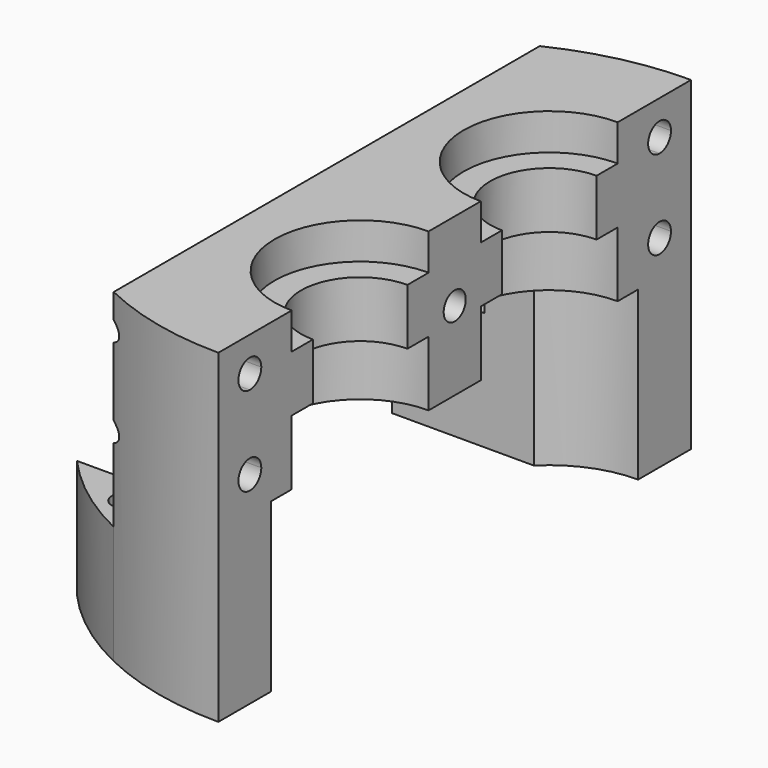
from build123d import *

# Parameters (mm, degrees)
F1_DEPTH      = 33
F3_DEPTH      = 12
F6_DEPTH      = 35.361679775
F7_R          = 6
F8_DEPTH      = 17.001
F9_W          = 4.1692499071
F9_H          = 40.0000885129
F10_DEPTH     = 8
F11_R         = 1.4
F12_DEPTH     = 35.361679775
F10_FACE2_W   = 4.1692499071
F10_FACE2_H   = 40.0000885129
F14_DEPTH     = 33.001
F15_W         = 2.69
F15_H         = 3.69
F15_H_2       = 6.6
F17_W         = 2.69
F17_H         = 6.6
F17_H_2       = 3.69
F20_DEPTH     = 33.001
F21_TEXT_SIZE = 11.6276503023
F22_DEPTH     = 1.69
F24_DEPTH     = 22.361679775


# Not quite as in the source:
# - Text() gives the source's letters only with a copy of the font that has no kerning and outlines rounded to 1/6400 em; it was checked with that copy


with BuildPart() as f1:
    # F0 (on Top) → F1 (new body)
    with BuildSketch(Plane.XY):
        with BuildLine():
            Line((-13, 27.0370116692), (13, 27.0370116692))
            ThreePointArc((13, 27.0370116692), (0, 30), (-13, 27.0370116692))
        make_face()
        with BuildLine():
            ThreePointArc((-13, -27.0370116692), (0, -30), (13, -27.0370116692))
            Line((13, -27.0370116692), (-13, -27.0370116692))
        make_face()
        with BuildLine():
            Line((13, -12), (6, -12))
            ThreePointArc((6, -12), (0, -18), (-6, -12))
            Line((-6, -12), (-13, -12))
            Line((-13, -12), (-13, -27.0370116692))
            Line((-13, -27.0370116692), (13, -27.0370116692))
            Line((13, -27.0370116692), (13, -12))
        make_face()
        with BuildLine():
            ThreePointArc((-6, -12), (0, -6), (6, -12))
            Line((6, -12), (13, -12))
            Line((13, -12), (13, 12))
            Line((13, 12), (6, 12))
            ThreePointArc((6, 12), (0, 6), (-6, 12))
            Line((-6, 12), (-13, 12))
            Line((-13, 12), (-13, -12))
            Line((-13, -12), (-6, -12))
        make_face()
        with BuildLine():
            Line((6, 12), (13, 12))
            Line((13, 12), (13, 27.0370116692))
            Line((13, 27.0370116692), (-13, 27.0370116692))
            Line((-13, 27.0370116692), (-13, 12))
            Line((-13, 12), (-6, 12))
            ThreePointArc((-6, 12), (0, 18), (6, 12))
        make_face()
    extrude(amount=F1_DEPTH)

    # F2 (on Top) → F3 (join)
    with BuildSketch(Plane.XY):
        with BuildLine():
            Line((-12.8831444308, 20), (22.360679775, 20))
            ThreePointArc((22.360679775, 20), (0, 30), (-22.360679775, 20))
            Line((-22.360679775, 20), (-12.8831444308, 20))
        make_face()
        with BuildLine():
            ThreePointArc((-22.360679775, -20), (0, -30), (22.360679775, -20))
            Line((22.360679775, -20), (-12.8831444308, -20))
            Line((-12.8831444308, -20), (-22.360679775, -20))
        make_face()
    extrude(amount=F3_DEPTH)

    # F5 (on face) → F6 (cut, through all)
    with BuildSketch(Plane(origin=(-13, 0, 0), x_dir=(0, -1, 0), z_dir=(-1, 0, 0))):
        Polygon((-20, 12), (-20, 0), (20, 0), (20, 12), (20, 17), (-20, 17), align=None)
    extrude(amount=-F6_DEPTH, mode=Mode.SUBTRACT)

    # F7 (on face) → F8 (cut, through all)
    with BuildSketch(Plane(origin=(0, 0, 17), x_dir=(1, 0, 0), z_dir=(0, 0, -1))):
        with BuildLine():
            ThreePointArc((-7.9664358404, 20), (-4.3314569928, 1.5739470403), (11.29, 12))
            ThreePointArc((11.29, 12), (10.4260529597, 16.3314569928), (7.9664358404, 20))
            Line((7.9664358404, 20), (-7.9664358404, 20))
        make_face()
        with Locations((0, 12)):
            Circle(F7_R, mode=Mode.SUBTRACT)
        with Locations((0, -12)):
            Circle(F7_R)
        with Locations((0, 12)):
            Circle(F7_R)
        with BuildLine():
            Line((-7.9664358404, 20), (7.9664358404, 20))
            ThreePointArc((7.9664358404, 20), (0, 23.29), (-7.9664358404, 20))
        make_face()
        with BuildLine():
            ThreePointArc((-7.9664358404, -20), (0, -23.29), (7.9664358404, -20))
            Line((7.9664358404, -20), (-7.9664358404, -20))
        make_face()
    extrude(amount=F8_DEPTH, mode=Mode.SUBTRACT)

    # F9 (on face) → F10 (join)
    with BuildSketch(Plane.XY.offset(33)):
        with Locations((10.915457271, 0)):
            Rectangle(F9_W, F9_H)
    extrude(amount=F10_DEPTH)

    # F11 (on face) → F12 (cut, through all)
    with BuildSketch(Plane.YZ.offset(13)):
        with Locations((-16.0000442564, 36)):
            Circle(F11_R)
        with Locations((15.9999557436, 36)):
            Circle(F11_R)
    extrude(amount=-F12_DEPTH, mode=Mode.SUBTRACT)

    # F4 (on face) + F10_face2 (on face) → F14 (cut, through all)
    with BuildSketch(Plane.XY.offset(33)):
        with BuildLine():
            Line((0, 36.6020798683), (0, 35.8893685043))
            Line((0, 35.8893685043), (0, 33.0385304987))
            Line((0, 33.0385304987), (0, 30))
            ThreePointArc((0, 30), (6.6666952054, 29.2498747867), (13, 27.0370116692))
            Line((13, 27.0370116692), (13, -27.0370116692))
            ThreePointArc((13, -27.0370116692), (6.6666952054, -29.2498747867), (0, -30))
            Line((0, -30), (0, -37.9473641515))
            Line((0, -37.9473641515), (28.5907108337, -37.9473641515))
            Line((28.5907108337, -37.9473641515), (28.5907108337, 36.6020798683))
            Line((28.5907108337, 36.6020798683), (0, 36.6020798683))
        make_face()
        with BuildLine():
            ThreePointArc((13, 27.0370116692), (6.6666952054, 29.2498747867), (0, 30))
            Line((0, 30), (0, 18))
            ThreePointArc((0, 18), (4.2426406871, 16.2426406871), (6, 12))
            ThreePointArc((6, 12), (4.2426406871, 7.7573593129), (0, 6))
            Line((0, 6), (0, -6))
            ThreePointArc((0, -6), (4.2426406871, -7.7573593129), (6, -12))
            ThreePointArc((6, -12), (4.2426406871, -16.2426406871), (0, -18))
            Line((0, -18), (0, -30))
            ThreePointArc((0, -30), (6.6666952054, -29.2498747867), (13, -27.0370116692))
            Line((13, -27.0370116692), (13, 27.0370116692))
        make_face()
    with BuildSketch(Plane(origin=(10.915457271, 0, 41), x_dir=(1, 0, 0), z_dir=(0, 0, 1))):
        Rectangle(F10_FACE2_W, F10_FACE2_H)
    extrude(amount=-F14_DEPTH, mode=Mode.SUBTRACT)

    # F15 (on face) → F16 (revolve, cut)
    with BuildSketch(Plane.YZ):
        with Locations((19.345, 31.155)):
            Rectangle(F15_W, F15_H)
        with Locations((19.345, 20.3)):
            Rectangle(F15_W, F15_H_2)
    revolve(axis=Axis((0, 12, 24.0890203007), (0, 0, -1)), mode=Mode.SUBTRACT)

    # F17 (on face) → F18 (revolve, cut)
    with BuildSketch(Plane.YZ):
        with Locations((-4.655, 20.3)):
            Rectangle(F17_W, F17_H)
        with Locations((-4.655, 31.155)):
            Rectangle(F17_W, F17_H_2)
    revolve(axis=Axis((0, -12, 20.3), (0, 0, -1)), mode=Mode.SUBTRACT)

    # F19 (on face) → F20 (cut, through all)
    with BuildSketch(Plane.XY.offset(33)):
        with BuildLine():
            ThreePointArc((-13.8336468603, 22.983035), (-16.0528856759, 23.9022738155), (-15.1336468603, 21.683035))
            Line((-15.1336468603, 21.683035), (-15.1336468603, 22.983035))
            Line((-15.1336468603, 22.983035), (-13.8336468603, 22.983035))
        make_face()
        with BuildLine():
            Line((-15.1336468603, 22.983035), (-15.1336468603, 21.683035))
            ThreePointArc((-15.1336468603, 21.683035), (-14.2144080448, 22.0637961845), (-13.8336468603, 22.983035))
            Line((-13.8336468603, 22.983035), (-15.1336468603, 22.983035))
        make_face()
        with BuildLine():
            Line((-15.1336468603, -22.983035), (-15.1336468603, -21.683035))
            ThreePointArc((-15.1336468603, -21.683035), (-16.0528856759, -23.9022738155), (-13.8336468603, -22.983035))
            Line((-13.8336468603, -22.983035), (-15.1336468603, -22.983035))
        make_face()
        with BuildLine():
            ThreePointArc((-13.8336468603, -22.983035), (-14.2144080448, -22.0637961845), (-15.1336468603, -21.683035))
            Line((-15.1336468603, -21.683035), (-15.1336468603, -22.983035))
            Line((-15.1336468603, -22.983035), (-13.8336468603, -22.983035))
        make_face()
    extrude(amount=-F20_DEPTH, mode=Mode.SUBTRACT)

    # F21 (on face) → F22 (cut)
    with BuildSketch(Plane(origin=(-13, 0, 0), x_dir=(0, -1, 0), z_dir=(-1, 0, 0))):
        with Locations((-22.959158886, 20.4480122775)):
            Text('ICEMAN', F21_TEXT_SIZE, font='Open Sans', font_style=FontStyle.BOLD, text_align=(TextAlign.LEFT, TextAlign.BOTTOM))
    extrude(amount=-F22_DEPTH, mode=Mode.SUBTRACT)

    # F23 (on face) → F24 (cut, through all)
    with BuildSketch(Plane.YZ):
        with BuildLine():
            ThreePointArc((26, 21.95), (24.9746951673, 21.5253048327), (24.55, 20.5))
            Line((24.55, 20.5), (26, 20.5))
            Line((26, 20.5), (26, 21.95))
        make_face()
        with BuildLine():
            Line((26, 20.5), (24.55, 20.5))
            ThreePointArc((24.55, 20.5), (26, 19.05), (27.45, 20.5))
            ThreePointArc((27.45, 20.5), (27.0253048327, 21.5253048327), (26, 21.95))
            Line((26, 21.95), (26, 20.5))
        make_face()
        with BuildLine():
            ThreePointArc((-26, 21.95), (-27.0253048327, 19.4746951673), (-24.55, 20.5))
            Line((-24.55, 20.5), (-26, 20.5))
            Line((-26, 20.5), (-26, 21.95))
        make_face()
        with BuildLine():
            Line((-26, 20.5), (-24.55, 20.5))
            ThreePointArc((-24.55, 20.5), (-24.9746951673, 21.5253048327), (-26, 21.95))
            Line((-26, 21.95), (-26, 20.5))
        make_face()
        with BuildLine():
            ThreePointArc((-1.4, 25), (0, 23.6), (1.4, 25))
            Line((1.4, 25), (0, 25))
            Line((0, 25), (-1.4, 25))
        make_face()
        with BuildLine():
            Line((0, 25), (1.4, 25))
            ThreePointArc((1.4, 25), (0, 26.4), (-1.4, 25))
            Line((-1.4, 25), (0, 25))
        make_face()
        with BuildLine():
            ThreePointArc((24.55, 29.5), (24.9746951673, 28.4746951673), (26, 28.05))
            Line((26, 28.05), (26, 29.5))
            Line((26, 29.5), (24.55, 29.5))
        make_face()
        with BuildLine():
            Line((26, 29.5), (26, 28.05))
            ThreePointArc((26, 28.05), (27.0253048327, 28.4746951673), (27.45, 29.5))
            ThreePointArc((27.45, 29.5), (26, 30.95), (24.55, 29.5))
            Line((24.55, 29.5), (26, 29.5))
        make_face()
        with BuildLine():
            ThreePointArc((-24.55, 29.5), (-27.0253048327, 30.5253048327), (-26, 28.05))
            Line((-26, 28.05), (-26, 29.5))
            Line((-26, 29.5), (-24.55, 29.5))
        make_face()
        with BuildLine():
            Line((-26, 29.5), (-26, 28.05))
            ThreePointArc((-26, 28.05), (-24.9746951673, 28.4746951673), (-24.55, 29.5))
            Line((-24.55, 29.5), (-26, 29.5))
        make_face()
    extrude(amount=-F24_DEPTH, mode=Mode.SUBTRACT)


solid = f1.part
